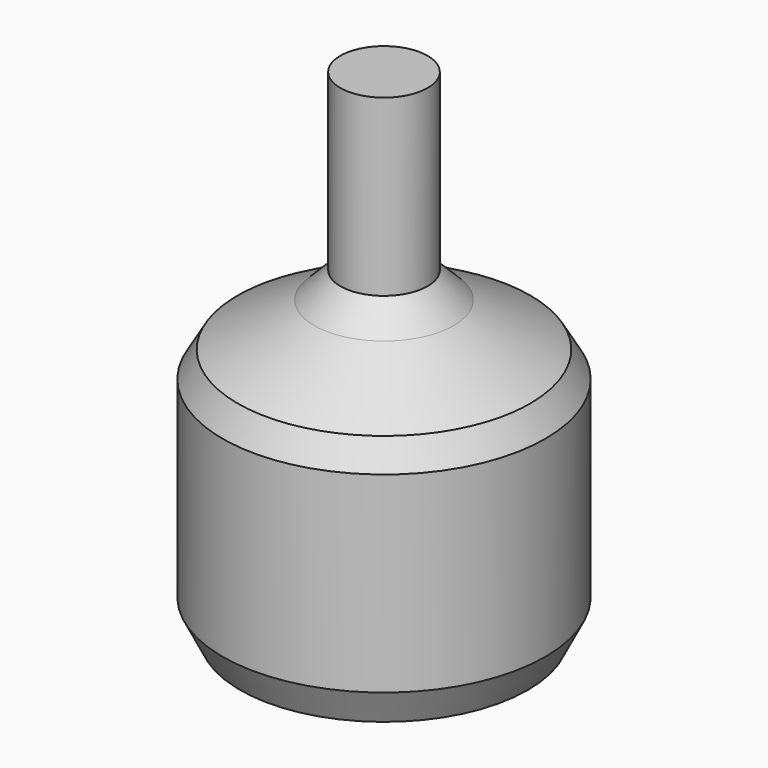
from build123d import *

# Parameters (mm, degrees)
F5_R       = 8.25
F6_R       = 9.25
F11_FACE_R = 9.25
F7_R       = 9.25
F12_FACE_R = 9.25
F9_R       = 4
F13_FACE_R = 4
F8_R       = 2.5
F14_FACE_R = 2.5
F10_R      = 2.5
F16_SIZE   = 1
F17_R      = 3
F18_DEPTH  = 2


with BuildPart() as f11:
    # F5 (on Top) → F11 section 0
    with BuildSketch(Plane.XY):
        Circle(F5_R)
    # F6 (on offset) → F11 section 1
    with BuildSketch(Plane.XY.offset(2)):
        Circle(F6_R)
    loft()

    # F11_face (on face) → F12 section 0
    with BuildSketch(Plane.XY.offset(2)):
        Circle(F11_FACE_R)
    # F7 (on offset) → F12 section 1
    with BuildSketch(Plane.XY.offset(14)):
        Circle(F7_R)
    loft()

    # F12_face (on face) → F13 section 0
    with BuildSketch(Plane.XY.offset(14)):
        Circle(F12_FACE_R)
    # F9 (on offset) → F13 section 1
    with BuildSketch(Plane.XY.offset(17)):
        Circle(F9_R)
    loft()

    # F13_face (on face) → F14 section 0
    with BuildSketch(Plane.XY.offset(17)):
        Circle(F13_FACE_R)
    # F8 (on offset) → F14 section 1
    with BuildSketch(Plane.XY.offset(18.5)):
        Circle(F8_R)
    loft()

    # F14_face (on face) → F15 section 0
    with BuildSketch(Plane.XY.offset(18.5)):
        Circle(F14_FACE_R)
    # F10 (on offset) → F15 section 1
    with BuildSketch(Plane.XY.offset(28.5)):
        Circle(F10_R)
    loft()

    # F16
    f16_edges = [f11.edges().sort_by_distance(p)[0] for p in [
        (-9.25, 0, 14),
    ]]
    chamfer(f16_edges, length=F16_SIZE)

    # F17 (on Top) → F18 (cut)
    with BuildSketch(Plane.XY):
        Circle(F17_R)
    extrude(amount=F18_DEPTH, mode=Mode.SUBTRACT)


solid = f11.part
